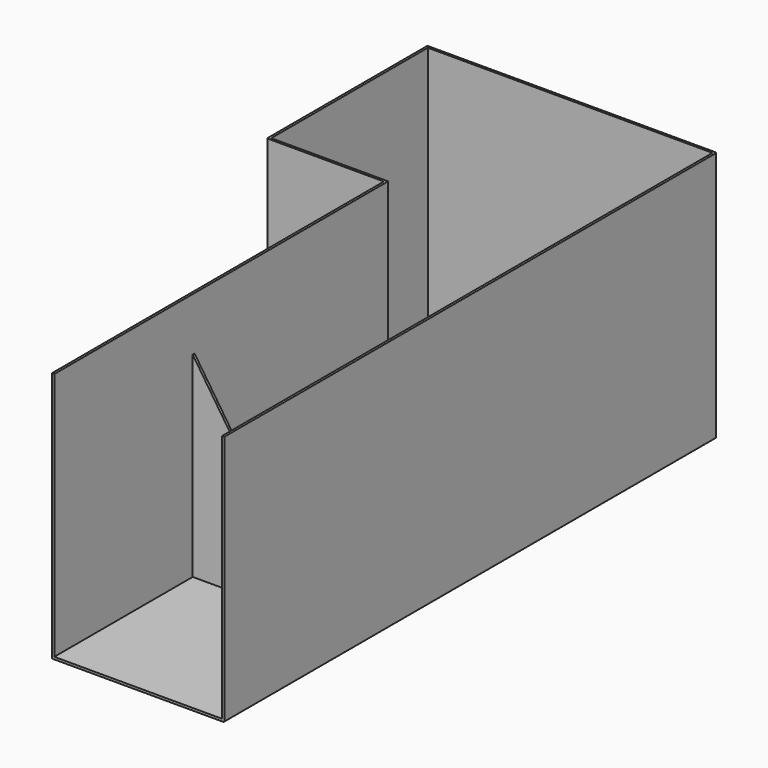
from build123d import *

# Parameters (mm, degrees)
F1_DEPTH  = 426
F3_DEPTH  = 4
F4_R      = 2
F7_DEPTH  = 4
F8_DEPTH  = 4
F11_DEPTH = 4


# Not quite as in the source:
# - a feature names something its author has since deleted; it is built from what else it names


with BuildPart() as f1:
    # F0 (on Top) → F1 (new body)
    with BuildSketch(Plane.XY):
        Polygon((495, 0), (0, 0), (0, -343), (200, -343), (200, -1053), (204, -1053), (204, -339), (4, -339), (4, -4), (491, -4), (491, -1053), (495, -1053), align=None)
    extrude(amount=F1_DEPTH)

    # F2 (on Top) → F3 (join)
    with BuildSketch(Plane.XY):
        Polygon((0, -343), (200, -343), (199.9874711037, -1053), (495, -1053), (495, 0), (0, 0), align=None)
    extrude(amount=-F3_DEPTH)

    # F4
    f4_edges = [f1.edges().sort_by_distance(p)[0] for p in [
        (100, -343, -4),
        (0, -171.5, -4),
        (247.5, 0, -4),
        (0, -343, 211),
        (0, 0, 211),
        (495, 0, 211),
        (199.993736, -698, -4),
        (495, -526.5, -4),
    ]]
    fillet(f4_edges, radius=F4_R)

    # F6 (on offset) → F7 (join)
    with BuildSketch(Plane.XZ.offset(753)):
        Polygon((426, 0), (204, 335), (204, 0), align=None)
    extrude(amount=F7_DEPTH)

    # F6 (on offset) → F8 (join)
    with BuildSketch(Plane.XZ.offset(753)):
        Polygon((426, 0), (204, 335), (204, 0), align=None)
    extrude(amount=F8_DEPTH)

    # F10 (on offset) → F11 (join)
    with BuildSketch(Plane.XZ.offset(153)):
        Polygon((491, 335), (269, 0), (491, 0), align=None)
    extrude(amount=F11_DEPTH)


solid = f1.part
